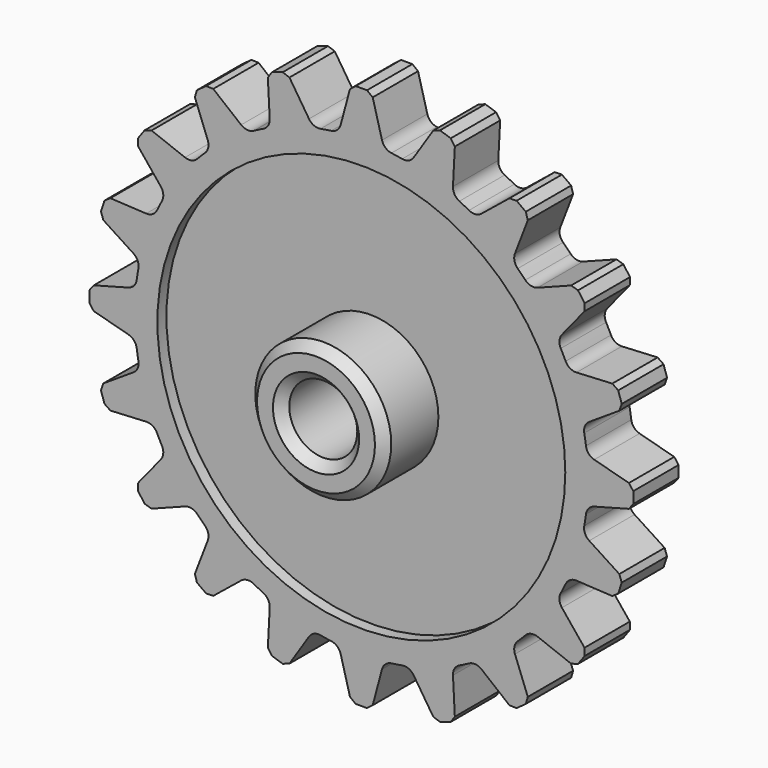
from build123d import *

# Parameters (mm, degrees)
F0_R            = 100
F1_DEPTH        = 25
F3_DEPTH        = 25
F3_COPIES_COUNT = 20
F4_SIZE         = 2
F5_R            = 5
F6_R            = 90
F7_DEPTH        = 5
F8_R            = 30
F9_DEPTH        = 30
F10_R           = 15
F11_DEPTH       = 50
F12_SIZE        = 4


# Not quite as in the source:
# - a pattern or mirror of a feature is missing from the dataset's text; its kind, count and spacing are read off the source's solid


with BuildPart() as f1:
    # F0 (on Front) → F1 (new body)
    with BuildSketch(Plane.XZ):
        Circle(F0_R)
    extrude(amount=F1_DEPTH)

    # F2 (on Front) → F3 (join)
    with BuildSketch(Plane.XZ):
        Polygon((-4.5, 120), (-9.9931095726, 99.4994359837), (9.9931095726, 99.4994359837), (4.5, 120), align=None)
    f3 = extrude(amount=F3_DEPTH)

    # F3_copies: F3 ×20 about axis
    f3_copies_axis = Axis((0, 0, 0), (0, 1, 0))
    for i in range(1, F3_COPIES_COUNT):
        add(f3.rotate(f3_copies_axis, i * 360 / F3_COPIES_COUNT))

    # F4
    f4_edges = [f1.edges().sort_by_distance(p)[0] for p in [
        (4.5, -12.5, 120),
        (-4.5, -12.5, 120),
        (-32.802285, -12.5, 115.517358),
        (115.517358, -12.5, 32.802285),
        (120, -12.5, 4.5),
        (120, -12.5, -4.5),
        (115.517358, -12.5, -32.802285),
        (112.736205, -12.5, -41.361794),
        (99.727073, -12.5, -66.893654),
        (94.437006, -12.5, -74.174807),
        (74.174807, -12.5, -94.437006),
        (66.893654, -12.5, -99.727073),
        (41.361794, -12.5, -112.736205),
        (32.802285, -12.5, -115.517358),
        (4.5, -12.5, -120),
        (-4.5, -12.5, -120),
        (-32.802285, -12.5, -115.517358),
        (-41.361794, -12.5, -112.736205),
        (-66.893654, -12.5, -99.727073),
        (-74.174807, -12.5, -94.437006),
        (-94.437006, -12.5, -74.174807),
        (-99.727073, -12.5, -66.893654),
        (-112.736205, -12.5, -41.361794),
        (-115.517358, -12.5, -32.802285),
        (-120, -12.5, -4.5),
        (-120, -12.5, 4.5),
        (-115.517358, -12.5, 32.802285),
        (-112.736205, -12.5, 41.361794),
        (-99.727073, -12.5, 66.893654),
        (-94.437006, -12.5, 74.174807),
        (-74.174807, -12.5, 94.437006),
        (-66.893654, -12.5, 99.727073),
        (32.802285, -12.5, 115.517358),
        (41.361794, -12.5, 112.736205),
        (66.893654, -12.5, 99.727073),
        (74.174807, -12.5, 94.437006),
        (94.437006, -12.5, 74.174807),
        (99.727073, -12.5, 66.893654),
        (112.736205, -12.5, 41.361794),
        (-41.361794, -12.5, 112.736205),
    ]]
    chamfer(f4_edges, length=F4_SIZE)

    # F5
    f5_edges = [f1.edges().sort_by_distance(p)[0] for p in [
        (9.99311, -12.5, 99.499436),
        (-9.99311, -12.5, 99.499436),
        (97.717628, -12.5, 21.243005),
        (99.499436, -12.5, 9.99311),
        (91.541546, -12.5, 40.251029),
        (86.370537, -12.5, 50.399706),
        (99.499436, -12.5, -9.99311),
        (97.717628, -12.5, -21.243005),
        (74.622932, -12.5, 66.568897),
        (66.568897, -12.5, 74.622932),
        (91.541546, -12.5, -40.251029),
        (86.370537, -12.5, -50.399706),
        (50.399706, -12.5, 86.370537),
        (40.251029, -12.5, 91.541546),
        (74.622932, -12.5, -66.568897),
        (66.568897, -12.5, -74.622932),
        (21.243005, -12.5, 97.717628),
        (50.399706, -12.5, -86.370537),
        (40.251029, -12.5, -91.541546),
        (-21.243005, -12.5, 97.717628),
        (21.243005, -12.5, -97.717628),
        (9.99311, -12.5, -99.499436),
        (-40.251029, -12.5, 91.541546),
        (-50.399706, -12.5, 86.370537),
        (-9.99311, -12.5, -99.499436),
        (-21.243005, -12.5, -97.717628),
        (-66.568897, -12.5, 74.622932),
        (-74.622932, -12.5, 66.568897),
        (-40.251029, -12.5, -91.541546),
        (-50.399706, -12.5, -86.370537),
        (-86.370537, -12.5, 50.399706),
        (-91.541546, -12.5, 40.251029),
        (-66.568897, -12.5, -74.622932),
        (-74.622932, -12.5, -66.568897),
        (-97.717628, -12.5, 21.243005),
        (-99.499436, -12.5, 9.99311),
        (-86.370537, -12.5, -50.399706),
        (-91.541546, -12.5, -40.251029),
        (-99.499436, -12.5, -9.99311),
        (-97.717628, -12.5, -21.243005),
    ]]
    fillet(f5_edges, radius=F5_R)

    # F6 (on face) → F7 (cut)
    with BuildSketch(Plane.XZ.offset(25)):
        Circle(F6_R)
    extrude(amount=-F7_DEPTH, mode=Mode.SUBTRACT)

    # F8 (on face) → F9 (join)
    with BuildSketch(Plane.XZ.offset(20)):
        Circle(F8_R)
    extrude(amount=F9_DEPTH)

    # F10 (on face) → F11 (cut, through all)
    with BuildSketch(Plane.XZ.offset(50)):
        Circle(F10_R)
    extrude(amount=-F11_DEPTH, mode=Mode.SUBTRACT)

    # F12
    f12_edges = [f1.edges().sort_by_distance(p)[0] for p in [
        (-30, -50, 0),
        (-15, -50, 0),
    ]]
    chamfer(f12_edges, length=F12_SIZE)


solid = f1.part
